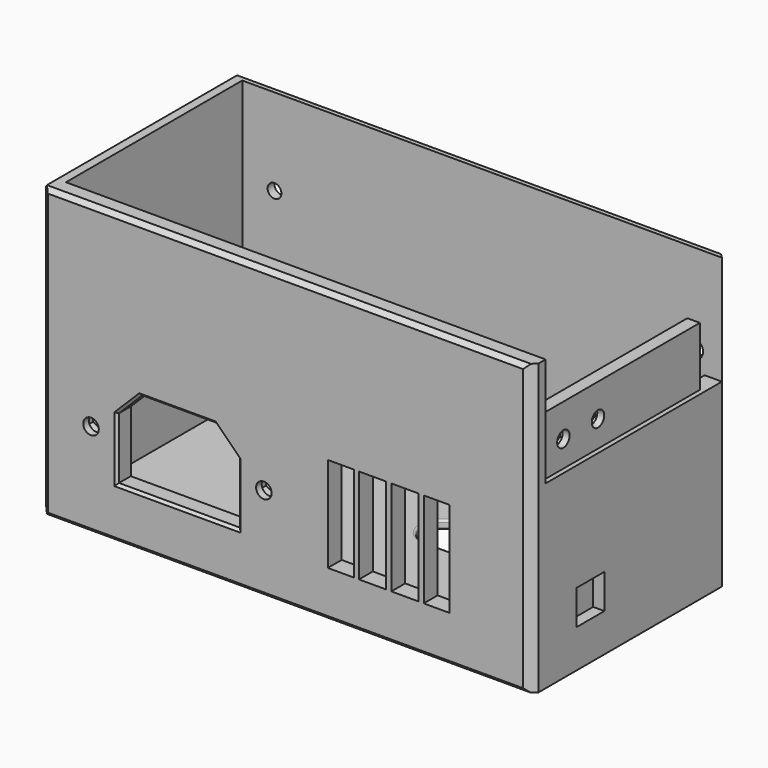
from build123d import *

# Parameters (mm, degrees)
F7_W      = 57
F7_H      = 65
F8_DEPTH  = 3
F6_W      = 114
F6_H      = 57
F6_W_2    = 30
F6_H_2    = 10
F9_DEPTH  = 2
F10_R     = 4.99999
F5_W      = 57
F5_H      = 53.4
F5_R      = 1.8
F11_DEPTH = 4
F12_W     = 51
F12_H     = 25.25
F13_DEPTH = 1.1
F14_DEPTH = 4
F15_W     = 5
F15_H     = 25.25
F16_DEPTH = 4.1
F1_W      = 111
F1_H      = 65
F1_R      = 1.5
F1_W_2    = 8
F1_H_2    = 8
F1_R_2    = 1.6
F1_R_3    = 2.1
F17_DEPTH = 2
F19_SIZE  = 2
F20_SIZE  = 2
F18_W     = 111
F18_H     = 65
F18_R     = 1.8
F18_W_2   = 28.2
F18_H_2   = 22
F21_DEPTH = 4
F22_SIZE  = 2
F23_SIZE  = 2
F24_SIZE  = 0.99999
F25_SIZE  = 0.99999
F26_R     = 0.5
F27_W     = 1.2
F27_H     = 4
F28_DEPTH = 22
F29_SIZE  = 0.6
F31_DEPTH = 1.3
F33_DEPTH = 2.38
F35_DEPTH = 1.2
F36_W     = 8
F36_H     = 8
F37_DEPTH = 2.6


# Not quite as in the source:
# - a fillet or chamfer is up to 0.001 mm smaller than in the source, because OpenCascade refuses the exact size


with BuildPart() as f8:
    # F7 (on offset) → F8 (new body)
    with BuildSketch(Plane.YZ.offset(-111)):
        with Locations((-28.5, 72.5)):
            Rectangle(F7_W, F7_H)
    extrude(amount=-F8_DEPTH)

    # F6 (on offset) → F9 (join)
    with BuildSketch(Plane.XY.offset(40)):
        with Locations((-57, -28.5)):
            Rectangle(F6_W, F6_H)
        with Locations((-40, -20)):
            Rectangle(F6_W_2, F6_H_2, mode=Mode.SUBTRACT)
    extrude(amount=-F9_DEPTH)

    # F10 (radius 5 in the source; OpenCascade refuses exactly that, so slightly less here)
    f10_edges = [f8.edges().sort_by_distance(p)[0] for p in [
        (-25, -25, 39),
        (-55, -25, 39),
        (-55, -15, 39),
        (-25, -15, 39),
    ]]
    fillet(f10_edges, radius=F10_R)

    # F5 (on Right) → F11 (join)
    with BuildSketch(Plane.YZ):
        with Locations((-28.5, 66.7)):
            Rectangle(F5_W, F5_H)
        with Locations((-46.4825592935, 85.7889130712)):
            Circle(F5_R, mode=Mode.SUBTRACT)
        with Locations((-36.4768356085, 85.8261138201)):
            Circle(F5_R, mode=Mode.SUBTRACT)
    extrude(amount=-F11_DEPTH)

    # F12 (on face) → F13 (cut)
    with BuildSketch(Plane.YZ):
        with Locations((-27.5, 92.375)):
            Rectangle(F12_W, F12_H)
    extrude(amount=-F13_DEPTH, mode=Mode.SUBTRACT)

    # F14 (add): a face of the model
    f14_faces = [f8.faces().sort_by_distance(p)[0] for p in [
        (0, -28.7827981232, 59.796589178),
    ]]
    extrude(f14_faces, amount=-F14_DEPTH)

    # F15 (on face) → F16 (cut)
    with BuildSketch(Plane.YZ):
        with Locations((-4.5, 92.375)):
            Rectangle(F15_W, F15_H)
    extrude(amount=-F16_DEPTH, mode=Mode.SUBTRACT)

    # F1 (on offset) → F17 (join)
    with BuildSketch(Plane.XZ.offset(2)):
        with Locations((-55.5, 72.5)):
            Rectangle(F1_W, F1_H)
        with Locations((-93.9863845706, 48.0133742094)):
            Circle(F1_R, mode=Mode.SUBTRACT)
        with Locations((-19.4850880653, 47.9871667922)):
            Circle(F1_R, mode=Mode.SUBTRACT)
        with Locations((-7.9999973103, 68.4999966025)):
            Rectangle(F1_W_2, F1_H_2, mode=Mode.SUBTRACT)
        with Locations((-103.55, 84.9350020289)):
            Circle(F1_R_2, mode=Mode.SUBTRACT)
        with Locations((-6.4611095004, 84.4112932682)):
            Circle(F1_R_3, mode=Mode.SUBTRACT)
    extrude(amount=-F17_DEPTH)

    # F19
    f19_edges = [f8.edges().sort_by_distance(p)[0] for p in [
        (0, 0, 71.5),
    ]]
    chamfer(f19_edges, length=F19_SIZE)

    # F20
    f20_edges = [f8.edges().sort_by_distance(p)[0] for p in [
        (-114, 0, 71.5),
    ]]
    chamfer(f20_edges, length=F20_SIZE)

    # F18 (on offset) → F21 (join)
    with BuildSketch(Plane.XZ.offset(53)):
        with Locations((-55.5, 72.5)):
            Rectangle(F18_W, F18_H)
        with Locations((-102, 59.8)):
            Circle(F18_R, mode=Mode.SUBTRACT)
        Polygon((-96, 64.2), (-90.6, 69.6), (-73.4, 69.6), (-68, 64.2), (-68, 50), (-96, 50), align=None, mode=Mode.SUBTRACT)
        with Locations((-62, 59.8)):
            Circle(F18_R, mode=Mode.SUBTRACT)
        with Locations((-33.1, 59.8)):
            Rectangle(F18_W_2, F18_H_2, mode=Mode.SUBTRACT)
    extrude(amount=F21_DEPTH)

    # F22
    f22_edges = [f8.edges().sort_by_distance(p)[0] for p in [
        (0, -57, 71.5),
    ]]
    chamfer(f22_edges, length=F22_SIZE)

    # F23
    f23_edges = [f8.edges().sort_by_distance(p)[0] for p in [
        (-114, -57, 71.5),
    ]]
    chamfer(f23_edges, length=F23_SIZE)

    # F24 (size 1 in the source; OpenCascade refuses exactly that, so slightly less here)
    f24_edges = [f8.edges().sort_by_distance(p)[0] for p in [
        (-57, -57, 105),
        (-57, 0, 105),
        (-114, -28.5, 105),
    ]]
    chamfer(f24_edges, length=F24_SIZE)

    # F25 (size 1 in the source; OpenCascade refuses exactly that, so slightly less here)
    f25_edges = [f8.edges().sort_by_distance(p)[0] for p in [
        (-57, -57, 38),
        (-114, -28.5, 38),
    ]]
    chamfer(f25_edges, length=F25_SIZE)

    # F26
    f26_edges = [f8.edges().sort_by_distance(p)[0] for p in [
        (-40, -25, 38),
        (-53.535537, -23.535537, 38),
        (-40, -15, 38),
        (-26.464463, -16.464463, 38),
        (-26.464463, -16.464463, 40),
        (-53.535537, -23.535537, 40),
    ]]
    fillet(f26_edges, radius=F26_R)

    # F27 (on face) → F28 (join, through all)
    with BuildSketch(Plane.XY.offset(48.8)):
        with Locations((-33.1, -55)):
            Rectangle(F27_W, F27_H)
        with Locations((-40.6, -55)):
            Rectangle(F27_W, F27_H)
        with Locations((-25.6, -55)):
            Rectangle(F27_W, F27_H)
    extrude(amount=F28_DEPTH)

    # F29
    f29_edges = [f8.edges().sort_by_distance(p)[0] for p in [
        (-82, -57, 50),
        (-68, -57, 57.1),
        (-70.7, -57, 66.9),
        (-82, -57, 69.6),
        (-93.3, -57, 66.9),
        (-96, -57, 57.1),
    ]]
    chamfer(f29_edges, length=F29_SIZE)

    # F30 (on face) → F31 (cut)
    with BuildSketch(Plane(origin=(-4, 0, 0), x_dir=(0, -1, 0), z_dir=(-1, 0, 0))):
        Polygon((39.1768356085, 84.2672680933), (39.1768356085, 87.3849595469), (36.4768356085, 88.9438052737), (33.7768356085, 87.3849595469), (33.7768356085, 84.2672680933), (36.4768356085, 82.7084223665), align=None)
        Polygon((49.1825592935, 84.2300673443), (49.1825592935, 87.347758798), (46.4825592935, 88.9066045248), (43.7825592935, 87.347758798), (43.7825592935, 84.2300673443), (46.4825592935, 82.6712216175), align=None)
    extrude(amount=-F31_DEPTH, mode=Mode.SUBTRACT)

    # F32 (on face) → F33 (cut)
    with BuildSketch(Plane.XZ.offset(53)):
        Polygon((-64.7, 61.3588457268), (-64.7, 58.2411542732), (-62, 56.6823085464), (-59.3, 58.2411542732), (-59.3, 61.3588457268), (-62, 62.9176914536), align=None)
        Polygon((-104.7, 61.3588457268), (-104.7, 58.2411542732), (-102, 56.6823085464), (-99.3, 58.2411542732), (-99.3, 61.3588457268), (-102, 62.9176914536), align=None)
    extrude(amount=F33_DEPTH, mode=Mode.SUBTRACT)

    # F34 (on face) → F35 (cut)
    with BuildSketch(Plane.XZ.offset(2)):
        Polygon((-91.2863845706, 46.4545284826), (-91.2863845706, 49.5722199362), (-93.9863845706, 51.131065663), (-96.6863845706, 49.5722199362), (-96.6863845706, 46.4545284826), (-93.9863845706, 44.8956827558), align=None)
        Polygon((-16.7850880653, 46.4283210653), (-16.7850880653, 49.546012519), (-19.4850880653, 51.1048582458), (-22.1850880653, 49.546012519), (-22.1850880653, 46.4283210653), (-19.4850880653, 44.8694753385), align=None)
    extrude(amount=-F35_DEPTH, mode=Mode.SUBTRACT)

    # F36 (on face) → F37 (cut)
    with BuildSketch(Plane.YZ):
        with Locations((-40, 50.8261138201)):
            Rectangle(F36_W, F36_H)
    extrude(amount=-F37_DEPTH, mode=Mode.SUBTRACT)


solid = f8.part
